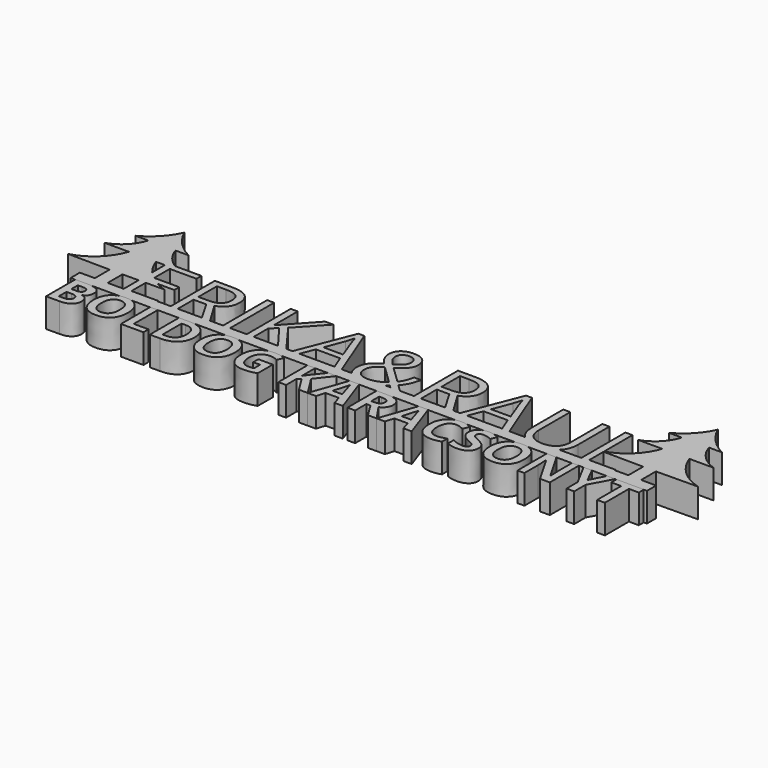
from build123d import *

# Parameters (mm, degrees)
F0_W         = 100
F0_H         = 2
F4_DEPTH     = 5
F1_TEXT_SIZE = 14.6837533004
F5_DEPTH     = 5
F2_TEXT_SIZE = 8.8522164214
F6_DEPTH     = 5


# Not quite as in the source:
# - a feature names something its author has since deleted; it is built from what else it names
# - Text() gives the source's letters only with a copy of the font that has no kerning and outlines rounded to 1/6400 em; it was checked with that copy


with BuildPart() as f4:
    # F0 (on Top) → F4 (new body)
    with BuildSketch(Plane.XY):
        with Locations((0, -0.0687486285)):
            Rectangle(F0_W, F0_H)
    extrude(amount=-F4_DEPTH)

    # F3 (on Top) + F1 (on Top) → F5 (join)
    with BuildSketch(Plane.XY):
        with BuildLine():
            ThreePointArc((-37.9231646657, 4.2189853266), (-41.6235133158, 6.295480724), (-43.9330533271, 9.8550366238))
            Line((-43.9330533271, 9.8550366238), (-39.7348068655, 9.8550366238))
            ThreePointArc((-39.7348068655, 9.8550366238), (-42.3527183825, 11.4605481491), (-43.9330533271, 14.093734324))
            Line((-43.9330533271, 14.093734324), (-41.6809134185, 14.093734324))
            ThreePointArc((-41.6809134185, 14.093734324), (-44.4008677148, 16.1335586025), (-46.2826507777, 18.9651530236))
            ThreePointArc((-46.2826507777, 18.9651530236), (-48.1644338405, 16.1335586025), (-50.8843881368, 14.093734324))
            Line((-50.8843881368, 14.093734324), (-48.6322482283, 14.093734324))
            ThreePointArc((-48.6322482283, 14.093734324), (-50.2125831729, 11.4605481491), (-52.8304946899, 9.8550366238))
            Line((-52.8304946899, 9.8550366238), (-48.6322482283, 9.8550366238))
            ThreePointArc((-48.6322482283, 9.8550366238), (-50.9417882396, 6.295480724), (-54.6421368896, 4.2189853266))
            Line((-54.6421368896, 4.2189853266), (-47.3919843614, 4.1369486087))
            Line((-47.3919843614, 4.1369486087), (-47.3919843614, 0))
            Line((-47.3919843614, 0), (-46.2826507777, 0))
            Line((-46.2826507777, 0), (-45.173317194, 0))
            Line((-45.173317194, 0), (-45.173317194, 4.1369486087))
            Line((-45.173317194, 4.1369486087), (-37.9231646657, 4.2189853266))
        make_face()
        with BuildLine():
            ThreePointArc((52.8304946899, 9.8550366238), (50.2125831729, 11.4605481491), (48.6322482283, 14.093734324))
            Line((48.6322482283, 14.093734324), (50.8843881368, 14.093734324))
            ThreePointArc((50.8843881368, 14.093734324), (48.1644338405, 16.1335586025), (46.2826507777, 18.9651530236))
            ThreePointArc((46.2826507777, 18.9651530236), (44.4008677148, 16.1335586025), (41.6809134185, 14.093734324))
            Line((41.6809134185, 14.093734324), (43.9330533271, 14.093734324))
            ThreePointArc((43.9330533271, 14.093734324), (42.3527183825, 11.4605481491), (39.7348068655, 9.8550366238))
            Line((39.7348068655, 9.8550366238), (43.9330533271, 9.8550366238))
            ThreePointArc((43.9330533271, 9.8550366238), (41.6235133158, 6.295480724), (37.9231646657, 4.2189853266))
            Line((37.9231646657, 4.2189853266), (45.173317194, 4.1369486087))
            Line((45.173317194, 4.1369486087), (45.173317194, 0))
            Line((45.173317194, 0), (46.2826507777, 0))
            Line((46.2826507777, 0), (47.3919843614, 0))
            Line((47.3919843614, 0), (47.3919843614, 4.1369486087))
            Line((47.3919843614, 4.1369486087), (54.6421368896, 4.2189853266))
            ThreePointArc((54.6421368896, 4.2189853266), (50.9417882396, 6.295480724), (48.6322482283, 9.8550366238))
            Line((48.6322482283, 9.8550366238), (52.8304946899, 9.8550366238))
        make_face()
    with BuildSketch(Plane.XY):
        with Locations((-43.8264149287, 0)):
            Text('ERIKA&RAUL', F1_TEXT_SIZE, font='Open Sans', text_align=(TextAlign.LEFT, TextAlign.BOTTOM))
    extrude(amount=-F5_DEPTH)


with BuildPart() as f6:
    # F2 (on Top) → F6 (new body)
    with BuildSketch(Plane.XY):
        with Locations((-50.0240133135, -7.3516160483)):
            Text('BOLDOG KARACSONYT', F2_TEXT_SIZE, font='Open Sans', font_style=FontStyle.BOLD, text_align=(TextAlign.LEFT, TextAlign.BOTTOM))
    extrude(amount=-F6_DEPTH)


solid = Compound([f4.part, f6.part])
